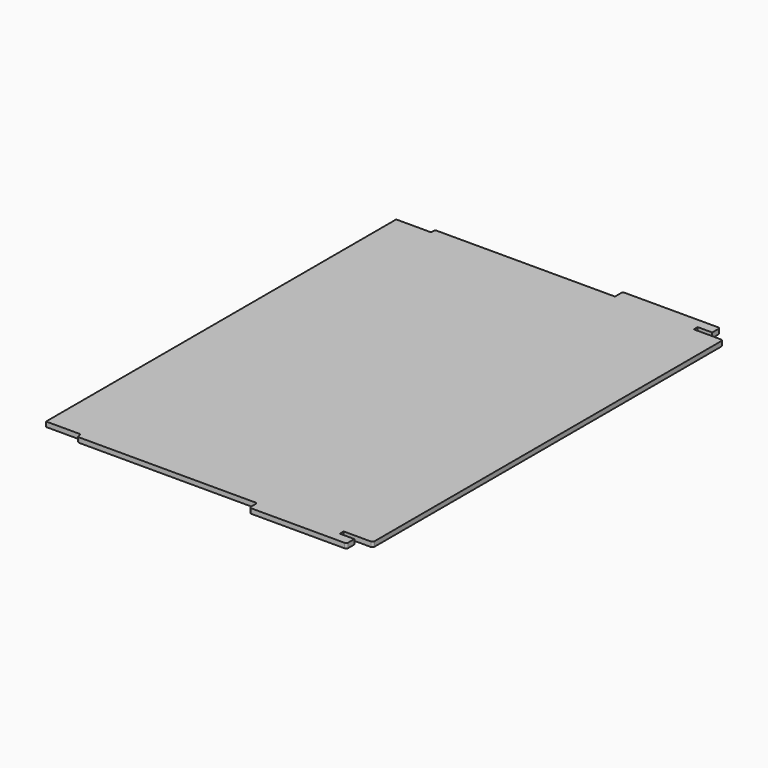
from build123d import *

# Parameters (mm, degrees)
F1_DEPTH = 5
F3_DEPTH = 25


with BuildPart() as f1:
    # F0 (on Top) → F1 (new body)
    with BuildSketch(Plane.XY):
        with BuildLine():
            Line((145, -225), (173, -225))
            ThreePointArc((173, -225), (174.4142135624, -224.4142135624), (175, -223))
            Line((175, -223), (175, 223))
            ThreePointArc((175, 223), (174.4142135624, 224.4142135624), (173, 225))
            Line((173, 225), (145, 225))
            Line((145, 225), (145, 230))
            Line((145, 230), (160, 230))
            Line((160, 230), (160, 238))
            ThreePointArc((160, 238), (159.4142135624, 239.4142135624), (158, 240))
            Line((158, 240), (62, 240))
            ThreePointArc((62, 240), (60.5857864376, 239.4142135624), (60, 238))
            Line((60, 238), (60, 230))
            Line((60, 230), (-123, 230))
            ThreePointArc((-123, 230), (-124.4142135624, 229.4142135624), (-125, 228))
            Line((-125, 228), (-125, 227))
            ThreePointArc((-125, 227), (-125.5857864376, 225.5857864376), (-127, 225))
            Line((-127, 225), (-173, 225))
            ThreePointArc((-173, 225), (-174.4142135624, 224.4142135624), (-175, 223))
            Line((-175, 223), (-175, -223))
            ThreePointArc((-175, -223), (-174.4142135624, -224.4142135624), (-173, -225))
            Line((-173, -225), (-127, -225))
            ThreePointArc((-127, -225), (-125.5857864376, -225.5857864376), (-125, -227))
            Line((-125, -227), (-125, -228))
            ThreePointArc((-125, -228), (-124.4142135624, -229.4142135624), (-123, -230))
            Line((-123, -230), (58, -230))
            ThreePointArc((58, -230), (59.4142135624, -230.5857864376), (60, -232))
            Line((60, -232), (60, -238))
            ThreePointArc((60, -238), (60.5857864376, -239.4142135624), (62, -240))
            Line((62, -240), (158, -240))
            ThreePointArc((158, -240), (159.4142135624, -239.4142135624), (160, -238))
            Line((160, -238), (160, -230))
            Line((160, -230), (145, -230))
            Line((145, -230), (145, -225))
        make_face()
    extrude(amount=F1_DEPTH)

    # F2 (on face) → F3 (cut)
    with BuildSketch(Plane.XY.offset(5)):
        with BuildLine():
            Line((-161, 225), (-161, 340.5782580579))
            Line((-161, 340.5782580579), (-227.952612991, 340.5782580579))
            Line((-227.952612991, 340.5782580579), (-227.952612991, -338.3395225013))
            Line((-227.952612991, -338.3395225013), (-161, -338.3395225013))
            Line((-161, -338.3395225013), (-161, -225))
            Line((-161, -225), (-173, -225))
            ThreePointArc((-173, -225), (-174.4142135624, -224.4142135624), (-175, -223))
            Line((-175, -223), (-175, 223))
            ThreePointArc((-175, 223), (-174.4142135624, 224.4142135624), (-173, 225))
            Line((-173, 225), (-161, 225))
        make_face()
        with BuildLine():
            Line((-161, -225), (-161, 225))
            Line((-161, 225), (-173, 225))
            ThreePointArc((-173, 225), (-174.4142135624, 224.4142135624), (-175, 223))
            Line((-175, 223), (-175, -223))
            ThreePointArc((-175, -223), (-174.4142135624, -224.4142135624), (-173, -225))
            Line((-173, -225), (-161, -225))
        make_face()
    extrude(amount=-F3_DEPTH, mode=Mode.SUBTRACT)


solid = f1.part
